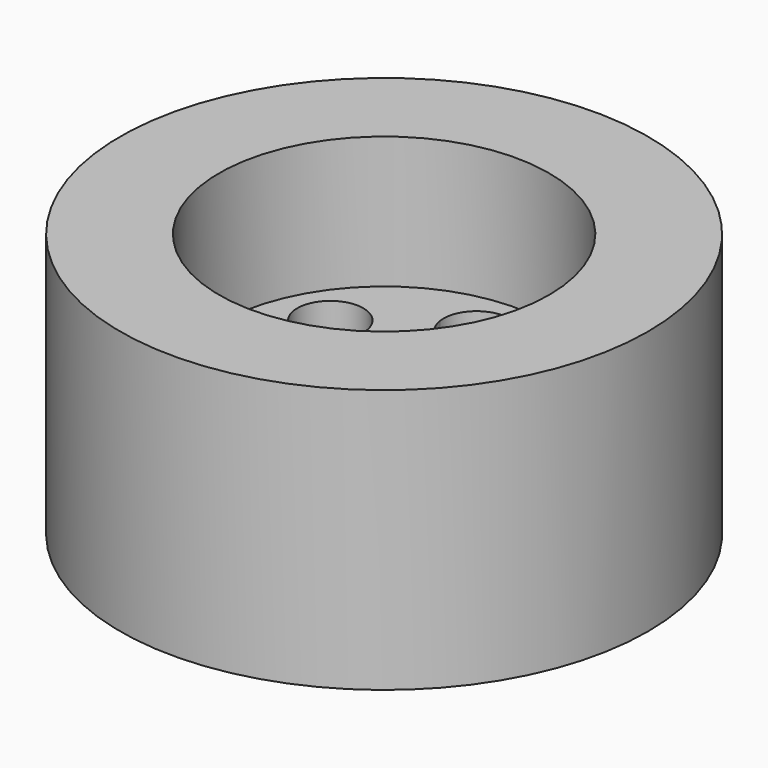
from build123d import *

# Parameters (mm, degrees)
F0_R     = 25.4
F0_R_2   = 2.3876
F1_DEPTH = 25.4
F2_R     = 15.875
F3_DEPTH = 12.7
F4_R     = 15.875
F4_R_2   = 6.35
F5_DEPTH = 6.35
F6_R     = 2.3876
F7_DEPTH = 12.701


with BuildPart() as f1:
    # F0 (on Top) → F1 (new body)
    with BuildSketch(Plane.XY):
        Circle(F0_R)
        Circle(F0_R_2, mode=Mode.SUBTRACT)
    extrude(amount=F1_DEPTH)

    # F2 (on face) → F3 (cut)
    with BuildSketch(Plane.XY.offset(25.4)):
        Circle(F2_R)
    extrude(amount=-F3_DEPTH, mode=Mode.SUBTRACT)

    # F4 (on face) → F5 (cut)
    with BuildSketch(Plane(origin=(0, 0, 0), x_dir=(1, 0, 0), z_dir=(0, 0, -1))):
        Circle(F4_R)
        Circle(F4_R_2, mode=Mode.SUBTRACT)
    extrude(amount=-F5_DEPTH, mode=Mode.SUBTRACT)

    # F6 (on face) → F7 (cut, through all)
    with BuildSketch(Plane.XY.offset(12.7)):
        with BuildLine():
            ThreePointArc((7.6596854017, 8.0508928571), (6.8740766425, 3.96875), (10.8021204383, 2.6080357143))
            ThreePointArc((10.8021204383, 2.6080357143), (9.6237072996, 5.55625), (7.6596854017, 8.0508928571))
        make_face()
        with BuildLine():
            ThreePointArc((7.6596854017, 8.0508928571), (9.6237072996, 5.55625), (10.8021204383, 2.6080357143))
            ThreePointArc((10.8021204383, 2.6080357143), (12.2525936337, 3.775918109), (12.7987072996, 5.55625))
            ThreePointArc((12.7987072996, 5.55625), (11.010223703, 8.4125058119), (7.6596854017, 8.0508928571))
        make_face()
        with BuildLine():
            ThreePointArc((12.7987072996, -5.55625), (12.2525936337, -3.775918109), (10.8021204383, -2.6080357143))
            ThreePointArc((10.8021204383, -2.6080357143), (9.6237072996, -5.55625), (7.6596854017, -8.0508928571))
            ThreePointArc((7.6596854017, -8.0508928571), (11.010223703, -8.4125058119), (12.7987072996, -5.55625))
        make_face()
        with BuildLine():
            ThreePointArc((7.6596854017, -8.0508928571), (9.6237072996, -5.55625), (10.8021204383, -2.6080357143))
            ThreePointArc((10.8021204383, -2.6080357143), (6.8740766425, -3.96875), (7.6596854017, -8.0508928571))
        make_face()
        with BuildLine():
            ThreePointArc((-3.1424350366, 10.6589285714), (0, 7.9375), (3.1424350366, 10.6589285714))
            ThreePointArc((3.1424350366, 10.6589285714), (0, 11.1125), (-3.1424350366, 10.6589285714))
        make_face()
        with BuildLine():
            ThreePointArc((-3.1424350366, 10.6589285714), (0, 11.1125), (3.1424350366, 10.6589285714))
            ThreePointArc((3.1424350366, 10.6589285714), (3.1668482945, 10.8851305222), (3.175, 11.1125))
            ThreePointArc((3.175, 11.1125), (-0.2273694778, 14.2793482945), (-3.1424350366, 10.6589285714))
        make_face()
        with BuildLine():
            ThreePointArc((3.175, -11.1125), (3.1668482945, -10.8851305222), (3.1424350366, -10.6589285714))
            ThreePointArc((3.1424350366, -10.6589285714), (0, -11.1125), (-3.1424350366, -10.6589285714))
            ThreePointArc((-3.1424350366, -10.6589285714), (-0.2273694778, -14.2793482945), (3.175, -11.1125))
        make_face()
        with BuildLine():
            ThreePointArc((-3.1424350366, -10.6589285714), (0, -11.1125), (3.1424350366, -10.6589285714))
            ThreePointArc((3.1424350366, -10.6589285714), (0, -7.9375), (-3.1424350366, -10.6589285714))
        make_face()
        with BuildLine():
            ThreePointArc((-6.4487072996, 5.55625), (-6.7674514877, 6.9427664035), (-7.6596854017, 8.0508928571))
            ThreePointArc((-7.6596854017, 8.0508928571), (-9.6237072996, 5.55625), (-10.8021204383, 2.6080357143))
            ThreePointArc((-10.8021204383, 2.6080357143), (-7.8433754085, 2.9273636659), (-6.4487072996, 5.55625))
        make_face()
        with BuildLine():
            ThreePointArc((-10.8021204383, 2.6080357143), (-9.6237072996, 5.55625), (-7.6596854017, 8.0508928571))
            ThreePointArc((-7.6596854017, 8.0508928571), (-12.3733379566, 7.14375), (-10.8021204383, 2.6080357143))
        make_face()
        with BuildLine():
            ThreePointArc((-10.8021204383, -2.6080357143), (-12.3733379566, -7.14375), (-7.6596854017, -8.0508928571))
            ThreePointArc((-7.6596854017, -8.0508928571), (-9.6237072996, -5.55625), (-10.8021204383, -2.6080357143))
        make_face()
        with BuildLine():
            ThreePointArc((-10.8021204383, -2.6080357143), (-9.6237072996, -5.55625), (-7.6596854017, -8.0508928571))
            ThreePointArc((-7.6596854017, -8.0508928571), (-6.7674514877, -6.9427664035), (-6.4487072996, -5.55625))
            ThreePointArc((-6.4487072996, -5.55625), (-7.8433754085, -2.9273636659), (-10.8021204383, -2.6080357143))
        make_face()
        Circle(F6_R)
    extrude(amount=-F7_DEPTH, mode=Mode.SUBTRACT)


solid = f1.part
